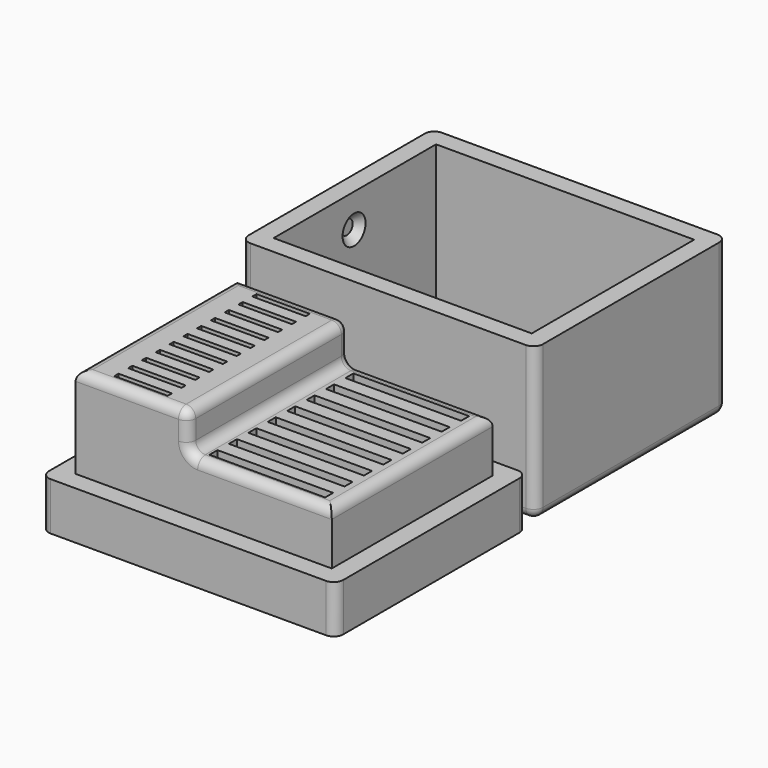
from build123d import *

# Parameters (mm, degrees)
F0_W      = 61.5
F0_H      = 50
F1_DEPTH  = 21
F2_W      = 61.5
F2_H      = 50
F2_W_2    = 53.5
F2_H_2    = 42
F3_DEPTH  = 11
F4_W      = 23.5
F4_H      = 42
F5_DEPTH  = 8
F6_W      = 11.15
F6_H      = 1.1
F7_DEPTH  = 7
F8_W      = 24.15
F8_H      = 2.1
F9_DEPTH  = 16
F10_F1_R  = 2
F10_F2_R  = 2
F11_W     = 61.5
F11_H     = 50
F12_DEPTH = 32
F13_W     = 53.9
F13_H     = 42.4
F14_DEPTH = 29
F15_R     = 2.5
F16_DEPTH = 1
F16_TAPER = 45
F17_R     = 3
F18_DEPTH = 1.5
F18_TAPER = 45
F19_R     = 2
F20_W     = 53.5
F20_H     = 42
F21_DEPTH = 2


with BuildPart() as f1:
    # F0 (on Top) → F1 (new body)
    with BuildSketch(Plane.XY):
        Rectangle(F0_W, F0_H)
    extrude(amount=F1_DEPTH)

    # F2 (on face) → F3 (cut)
    with BuildSketch(Plane.XY.offset(21)):
        Rectangle(F2_W, F2_H)
        Rectangle(F2_W_2, F2_H_2, mode=Mode.SUBTRACT)
    extrude(amount=-F3_DEPTH, mode=Mode.SUBTRACT)

    # F4 (on face) → F5 (join)
    with BuildSketch(Plane.XY.offset(21)):
        with Locations((-15, 0)):
            Rectangle(F4_W, F4_H)
    extrude(amount=F5_DEPTH)

    # F6 (on face) → F7 (cut)
    with BuildSketch(Plane.XY.offset(29)):
        with Locations((-15, 17.95)):
            Rectangle(F6_W, F6_H)
        with Locations((-15, 14.3500323179)):
            Rectangle(F6_W, F6_H)
        with Locations((-15, 10.7500646357)):
            Rectangle(F6_W, F6_H)
        with Locations((-15, 7.1500969536)):
            Rectangle(F6_W, F6_H)
        with Locations((-15, 3.5501292715)):
            Rectangle(F6_W, F6_H)
        with Locations((-15, -0.0498384107)):
            Rectangle(F6_W, F6_H)
        with Locations((-15, -3.6498060928)):
            Rectangle(F6_W, F6_H)
        with Locations((-15, -7.249773775)):
            Rectangle(F6_W, F6_H)
        with Locations((-15, -10.8497414571)):
            Rectangle(F6_W, F6_H)
        with Locations((-15, -14.4497091392)):
            Rectangle(F6_W, F6_H)
        with Locations((-15, -18.0496768214)):
            Rectangle(F6_W, F6_H)
    extrude(amount=-F7_DEPTH, mode=Mode.SUBTRACT)

    # F8 (on face) → F9 (cut)
    with BuildSketch(Plane.XY.offset(21)):
        with Locations((11.75, 17.45)):
            Rectangle(F8_W, F8_H)
        with Locations((11.6948562951, 12.4503040921)):
            Rectangle(F8_W, F8_H)
        with Locations((11.6397125903, 7.4506081841)):
            Rectangle(F8_W, F8_H)
        with Locations((11.5845688854, 2.4509122762)):
            Rectangle(F8_W, F8_H)
        with Locations((11.5294251805, -2.5487836317)):
            Rectangle(F8_W, F8_H)
        with Locations((11.4742814757, -7.5484795397)):
            Rectangle(F8_W, F8_H)
        with Locations((11.4191377708, -12.5481754476)):
            Rectangle(F8_W, F8_H)
        with Locations((11.3639940659, -17.5478713555)):
            Rectangle(F8_W, F8_H)
    extrude(amount=-F9_DEPTH, mode=Mode.SUBTRACT)

    # F10: fillet of radius 2 on 12 edges, made by hand

    # F10_f1
    f10_f1_edges = [f1.edges().sort_by_distance(p)[0] for p in [
        (-3.25, 0, 21),
    ]]
    fillet(f10_f1_edges, radius=F10_F1_R)

    # F10_f2
    f10_f2_edges = [f1.edges().sort_by_distance(p)[0] for p in [
        (-3.25, 0, 29),
        (26.75, 0, 21),
        (-26.75, 0, 29),
        (-30.75, -25, 5),
        (-30.75, 25, 5),
        (30.75, -25, 5),
        (30.75, 25, 5),
        (-15, -21, 29),
        (12.75, -21, 21),
        (12.75, 21, 21),
        (-15, 21, 29),
        (-2.6642135624, 21, 21.5857864376),
        (-2.6642135624, -21, 21.5857864376),
    ]]
    fillet(f10_f2_edges, radius=F10_F2_R)

    # F15 (on face) → F16 (join)
    with BuildSketch(Plane(origin=(-26.75, 0, 0), x_dir=(0, -1, 0), z_dir=(-1, 0, 0))):
        with Locations((0, 18.5)):
            Circle(F15_R)
    extrude(amount=F16_DEPTH, taper=F16_TAPER)

    # F20 (on face) → F21 (cut)
    with BuildSketch(Plane(origin=(0, 0, 0), x_dir=(1, 0, 0), z_dir=(0, 0, -1))):
        Rectangle(F20_W, F20_H)
    extrude(amount=-F21_DEPTH, mode=Mode.SUBTRACT)


with BuildPart() as f12:
    # F11 (on Top) → F12 (new body)
    with BuildSketch(Plane.XY):
        with Locations((-0.1928630173, 52.3866325617)):
            Rectangle(F11_W, F11_H)
    extrude(amount=F12_DEPTH)

    # F13 (on face) → F14 (cut)
    with BuildSketch(Plane.XY.offset(32)):
        with Locations((-0.1928630173, 52.3866325617)):
            Rectangle(F13_W, F13_H)
    extrude(amount=-F14_DEPTH, mode=Mode.SUBTRACT)

    # F17 (on face) → F18 (cut)
    with BuildSketch(Plane.YZ.offset(-27.1428630173)):
        with Locations((52.1866325617, 25)):
            Circle(F17_R)
    extrude(amount=-F18_DEPTH, taper=F18_TAPER, mode=Mode.SUBTRACT)

    # F19
    f19_edges = [f12.edges().sort_by_distance(p)[0] for p in [
        (-0.192863, 77.386633, 0),
        (-30.942863, 52.386633, 0),
        (-0.192863, 27.386633, 0),
        (30.557137, 52.386633, 0),
        (-30.942863, 77.386633, 16),
        (-30.942863, 27.386633, 16),
        (30.557137, 27.386633, 16),
        (30.557137, 77.386633, 16),
    ]]
    fillet(f19_edges, radius=F19_R)


solid = Compound([f1.part, f12.part])
